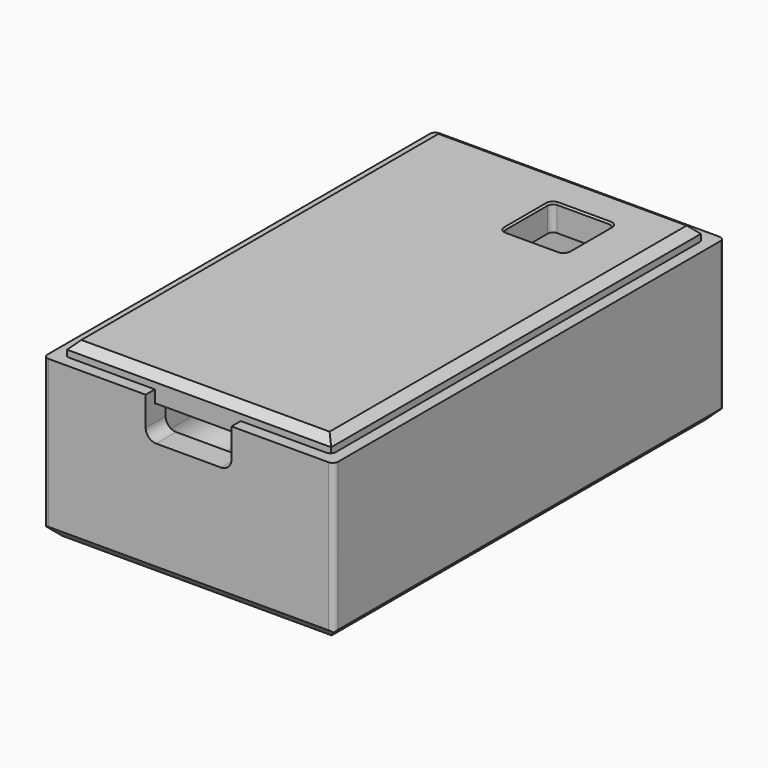
from build123d import *

# Parameters (mm, degrees)
F0_W      = 69.85
F0_H      = 117.475
F1_DEPTH  = 38.1
F2_T      = -6
F4_W      = 64.29375
F4_H      = 111.91875
F5_DEPTH  = 3.175
F6_R      = 1.190625
F7_DEPTH  = 6.35
F10_DEPTH = 1.7859375
F11_W     = 20.6375
F11_H     = 6.5167046964
F12_DEPTH = 9.525
F13_R     = 6.34999
F14_R     = 1.27
F15_SIZE  = 2.54
F16_R     = 1.27
F17_R     = 2.54
F18_R     = 1.27
F19_W     = 63.5
F19_H     = 111.125
F20_DEPTH = 6.35
F21_SIZE  = 1.905
F23_W     = 15.08125
F23_H     = 15.08125
F24_DEPTH = 25.4
F25_R     = 1.27
F26_R     = 0.79375
F27_DEPTH = 0.79375
F28_DEPTH = 0.79375
F29_SIZE  = 0.4
F30_R     = 3.460625
F30_R_2   = 2.460625
F31_DEPTH = 2.38125


# Not quite as in the source:
# - a fillet or chamfer is up to 0.001 mm smaller than in the source, because OpenCascade refuses the exact size


with BuildPart() as f1:
    # F0 (on Top) → F1 (new body)
    with BuildSketch(Plane.XY):
        Rectangle(F0_W, F0_H)
    extrude(amount=F1_DEPTH)

    # F2
    f2_openings = [f1.faces().sort_by_distance(p)[0] for p in [
        (0, 0, 38.1),
    ]]
    offset(amount=F2_T, openings=f2_openings)

    # F4 (on offset) → F5 (cut)
    with BuildSketch(Plane.XY.offset(38.1)):
        Rectangle(F4_W, F4_H)
    extrude(amount=-F5_DEPTH, mode=Mode.SUBTRACT)

    # F6 (on face) → F7 (join)
    with BuildSketch(Plane.XY.offset(6)):
        with BuildLine():
            Line((-28.925, -52.7375), (-13.685, -52.7375))
            ThreePointArc((-13.685, -52.7375), (-18.1486926547, -41.9611926547), (-28.925, -37.4975))
            Line((-28.925, -37.4975), (-28.925, -52.7375))
        make_face()
        with Locations((-22.165, -45.6)):
            Circle(F6_R, mode=Mode.SUBTRACT)
        with BuildLine():
            Line((-28.925, 52.7375), (-28.925, 37.4975))
            ThreePointArc((-28.925, 37.4975), (-18.1486926547, 41.9611926547), (-13.685, 52.7375))
            Line((-13.685, 52.7375), (-28.925, 52.7375))
        make_face()
        with Locations((-22.165, 45.6)):
            Circle(F6_R, mode=Mode.SUBTRACT)
        with BuildLine():
            Line((28.925, -52.7375), (28.925, -37.4975))
            ThreePointArc((28.925, -37.4975), (18.1486926547, -41.9611926547), (13.685, -52.7375))
            Line((13.685, -52.7375), (28.925, -52.7375))
        make_face()
        with Locations((22.165, -45.6)):
            Circle(F6_R, mode=Mode.SUBTRACT)
        with BuildLine():
            Line((28.925, 52.7375), (13.685, 52.7375))
            ThreePointArc((13.685, 52.7375), (18.1486926547, 41.9611926547), (28.925, 37.4975))
            Line((28.925, 37.4975), (28.925, 52.7375))
        make_face()
        with Locations((22.165, 45.6)):
            Circle(F6_R, mode=Mode.SUBTRACT)
    extrude(amount=F7_DEPTH)

    # F9 (on offset) → F10 (cut)
    with BuildSketch(Plane.XY.offset(12.35)):
        Polygon((-20.79, -47.9815698604), (-19.415, -45.6), (-20.79, -43.2184301396), (-23.54, -43.2184301396), (-24.915, -45.6), (-23.54, -47.9815698604), align=None)
        Polygon((20.79, -47.9815698604), (23.54, -47.9815698604), (24.915, -45.6), (23.54, -43.2184301396), (20.79, -43.2184301396), (19.415, -45.6), align=None)
        Polygon((-19.415, 45.6), (-20.79, 47.9815698604), (-23.54, 47.9815698604), (-24.915, 45.6), (-23.54, 43.2184301396), (-20.79, 43.2184301396), align=None)
        Polygon((23.54, 43.2184301396), (24.915, 45.6), (23.54, 47.9815698604), (20.79, 47.9815698604), (19.415, 45.6), (20.79, 43.2184301396), align=None)
    extrude(amount=-F10_DEPTH, mode=Mode.SUBTRACT)

    # F11 (on face) → F12 (cut)
    with BuildSketch(Plane.XY.offset(38.1)):
        with Locations((0, -55.4791476518)):
            Rectangle(F11_W, F11_H)
    extrude(amount=-F12_DEPTH, mode=Mode.SUBTRACT)

    # F13 (radius 6.35 in the source; OpenCascade refuses exactly that, so slightly less here)
    f13_edges = [f1.edges().sort_by_distance(p)[0] for p in [
        (-18.148693, 41.961193, 6),
        (0, 52.7375, 6),
        (18.148693, 41.961193, 6),
        (28.925, 0, 6),
        (18.148693, -41.961193, 6),
        (0, -52.7375, 6),
        (-18.148693, -41.961193, 6),
        (-28.925, 0, 6),
    ]]
    fillet(f13_edges, radius=F13_R)

    # F14
    f14_edges = [f1.edges().sort_by_distance(p)[0] for p in [
        (-28.925, -52.7375, 23.6375),
        (-28.925, 52.7375, 23.6375),
        (28.925, -52.7375, 23.6375),
        (28.925, 52.7375, 23.6375),
    ]]
    fillet(f14_edges, radius=F14_R)

    # F15
    f15_edges = [f1.edges().sort_by_distance(p)[0] for p in [
        (-34.925, 0, 0),
        (0, -58.7375, 0),
        (34.925, 0, 0),
        (0, 58.7375, 0),
    ]]
    chamfer(f15_edges, length=F15_SIZE)

    # F16
    f16_edges = [f1.edges().sort_by_distance(p)[0] for p in [
        (34.925, -58.7375, 20.32),
        (-34.925, -58.7375, 20.32),
        (-34.925, 58.7375, 20.32),
        (34.925, 58.7375, 20.32),
    ]]
    fillet(f16_edges, radius=F16_R)

    # F17
    f17_edges = [f1.edges().sort_by_distance(p)[0] for p in [
        (10.31875, -55.7375, 28.575),
        (-10.31875, -55.7375, 28.575),
    ]]
    fillet(f17_edges, radius=F17_R)

    # F18
    f18_edges = [f1.edges().sort_by_distance(p)[0] for p in [
        (32.146875, -55.959375, 36.5125),
        (32.146875, 55.959375, 36.5125),
        (-32.146875, 55.959375, 36.5125),
        (-32.146875, -55.959375, 36.5125),
    ]]
    fillet(f18_edges, radius=F18_R)

    # F26 (on face) → F27 (cut)
    with BuildSketch(Plane.XY.offset(34.925)):
        with Locations((30.1625, 53.4240681234)):
            Circle(F26_R)
        with Locations((30.1625, -53.4240681234)):
            Circle(F26_R)
        with Locations((-30.1625, -53.4240681234)):
            Circle(F26_R)
        with Locations((-30.1625, 53.4240681234)):
            Circle(F26_R)
    extrude(amount=-F27_DEPTH, mode=Mode.SUBTRACT)


with BuildPart() as f20:
    # F19 (on face) → F20 (new body)
    with BuildSketch(Plane.XY.offset(34.925)):
        Rectangle(F19_W, F19_H)
    extrude(amount=F20_DEPTH)

    # F21
    f21_edges = [f20.edges().sort_by_distance(p)[0] for p in [
        (0, 55.5625, 41.275),
        (-31.75, 0, 41.275),
        (0, -55.5625, 41.275),
        (31.75, 0, 41.275),
    ]]
    chamfer(f21_edges, length=F21_SIZE)

    # F23 (on offset) → F24 (cut)
    with BuildSketch(Plane.XY.offset(44.45)):
        with Locations((11.449375, 38.059375)):
            Rectangle(F23_W, F23_H)
    extrude(amount=-F24_DEPTH, mode=Mode.SUBTRACT)

    # F25
    f25_edges = [f20.edges().sort_by_distance(p)[0] for p in [
        (18.99, 45.6, 38.1),
        (3.90875, 45.6, 38.1),
        (3.90875, 30.51875, 38.1),
        (18.99, 30.51875, 38.1),
    ]]
    fillet(f25_edges, radius=F25_R)

    # F26 (on face) → F28 (cut)
    with BuildSketch(Plane.XY.offset(34.925)):
        with Locations((30.1625, 53.4240681234)):
            Circle(F26_R)
        with Locations((30.1625, -53.4240681234)):
            Circle(F26_R)
        with Locations((-30.1625, -53.4240681234)):
            Circle(F26_R)
        with Locations((-30.1625, 53.4240681234)):
            Circle(F26_R)
    extrude(amount=F28_DEPTH, mode=Mode.SUBTRACT)

    # F29
    f29_edges = [f20.edges().sort_by_distance(p)[0] for p in [
        (11.449375, 45.6, 41.275),
    ]]
    chamfer(f29_edges, length=F29_SIZE)


with BuildPart() as f31:
    # F30 (on face) → F31 (new body)
    with BuildSketch(Plane.XY.offset(12.35)):
        with Locations((-22.165, 45.6)):
            Circle(F30_R)
        with Locations((-22.165, 45.6)):
            Circle(F30_R_2, mode=Mode.SUBTRACT)
    extrude(amount=F31_DEPTH)


with BuildPart() as f31b:
    # F30 (on face) → F31, piece 2 (new body)
    with BuildSketch(Plane.XY.offset(12.35)):
        with Locations((22.165, 45.6)):
            Circle(F30_R)
        with Locations((22.165, 45.6)):
            Circle(F30_R_2, mode=Mode.SUBTRACT)
    extrude(amount=F31_DEPTH)


with BuildPart() as f31c:
    # F30 (on face) → F31, piece 3 (new body)
    with BuildSketch(Plane.XY.offset(12.35)):
        with Locations((-22.165, -45.6)):
            Circle(F30_R)
        with Locations((-22.165, -45.6)):
            Circle(F30_R_2, mode=Mode.SUBTRACT)
    extrude(amount=F31_DEPTH)


with BuildPart() as f31d:
    # F30 (on face) → F31, piece 4 (new body)
    with BuildSketch(Plane.XY.offset(12.35)):
        with Locations((22.165, -45.6)):
            Circle(F30_R)
        with Locations((22.165, -45.6)):
            Circle(F30_R_2, mode=Mode.SUBTRACT)
    extrude(amount=F31_DEPTH)


solid = Compound([f1.part, f20.part, f31.part, f31b.part, f31c.part, f31d.part])
